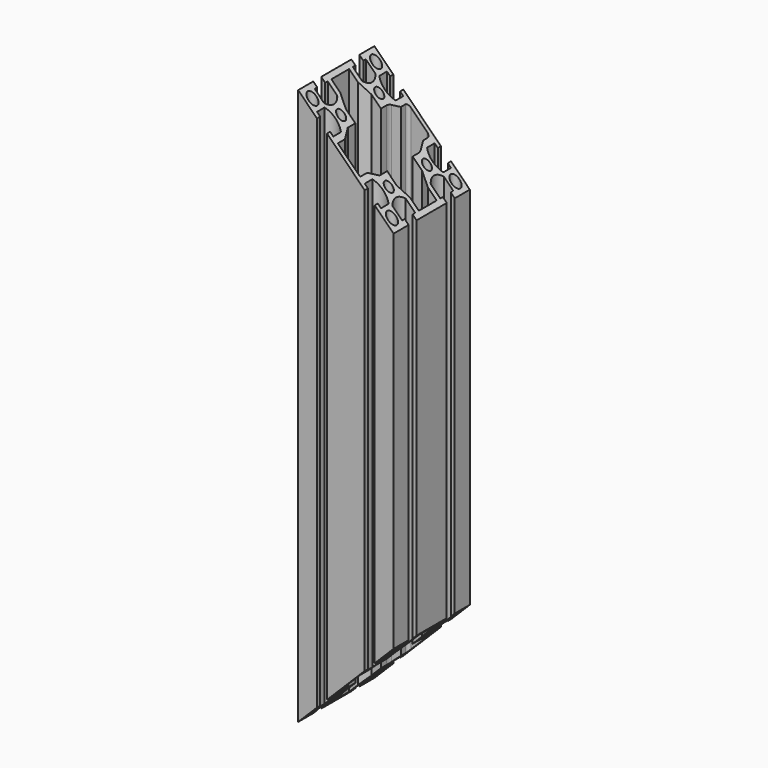
from build123d import *

# Parameters (mm, degrees)
F0_R     = 3
F0_R_2   = 2.5
F1_DEPTH = 350
F2_R     = 2
F3_R     = 7
F5_DEPTH = 60


# Not quite as in the source:
# - a feature names something its author has since deleted; it is built from what else it names


with BuildPart() as f1:
    # F0 (on Top) → F1 (new body)
    with BuildSketch(Plane.XY):
        with BuildLine():
            Line((18.15, -30), (30, -30))
            Line((30, -30), (30, -18.15))
            Line((30, -18.15), (27.5, -18.15))
            Line((27.5, -18.15), (27.5, -20.15))
            Line((27.5, -20.15), (21.5477069044, -20.15))
            ThreePointArc((21.5477069044, -20.15), (19.5, -15), (21.5477069044, -9.85))
            Line((21.5477069044, -9.85), (27.5, -9.85))
            Line((27.5, -9.85), (27.5, -11.85))
            Line((27.5, -11.85), (30, -11.85))
            Line((30, -11.85), (30, 11.85))
            Line((30, 11.85), (27.5, 11.85))
            Line((27.5, 11.85), (27.5, 9.85))
            Line((27.5, 9.85), (21.5477069044, 9.85))
            ThreePointArc((21.5477069044, 9.85), (19.5, 15), (21.5477069044, 20.15))
            Line((21.5477069044, 20.15), (27.5, 20.15))
            Line((27.5, 20.15), (27.5, 18.15))
            Line((27.5, 18.15), (30, 18.15))
            Line((30, 18.15), (30, 30))
            Line((30, 30), (18.15, 30))
            Line((18.15, 30), (18.15, 27.5))
            Line((18.15, 27.5), (20.15, 27.5))
            Line((20.15, 27.5), (20.15, 21.5477069044))
            ThreePointArc((20.15, 21.5477069044), (15, 19.5), (9.85, 21.5477069044))
            Line((9.85, 21.5477069044), (9.85, 27.5))
            Line((9.85, 27.5), (11.85, 27.5))
            Line((11.85, 27.5), (11.85, 30))
            Line((11.85, 30), (-11.85, 30))
            Line((-11.85, 30), (-11.85, 27.5))
            Line((-11.85, 27.5), (-9.85, 27.5))
            Line((-9.85, 27.5), (-9.85, 21.5477069044))
            ThreePointArc((-9.85, 21.5477069044), (-15, 19.5), (-20.15, 21.5477069044))
            Line((-20.15, 21.5477069044), (-20.15, 27.5))
            Line((-20.15, 27.5), (-18.15, 27.5))
            Line((-18.15, 27.5), (-18.15, 30))
            Line((-18.15, 30), (-30, 30))
            Line((-30, 30), (-30, 18.15))
            Line((-30, 18.15), (-27.5, 18.15))
            Line((-27.5, 18.15), (-27.5, 20.15))
            Line((-27.5, 20.15), (-21.5477069044, 20.15))
            ThreePointArc((-21.5477069044, 20.15), (-19.5, 15), (-21.5477069044, 9.85))
            Line((-21.5477069044, 9.85), (-27.5, 9.85))
            Line((-27.5, 9.85), (-27.5, 11.85))
            Line((-27.5, 11.85), (-30, 11.85))
            Line((-30, 11.85), (-30, -11.85))
            Line((-30, -11.85), (-27.5, -11.85))
            Line((-27.5, -11.85), (-27.5, -9.85))
            Line((-27.5, -9.85), (-21.5477069044, -9.85))
            ThreePointArc((-21.5477069044, -9.85), (-19.5, -15), (-21.5477069044, -20.15))
            Line((-21.5477069044, -20.15), (-27.5, -20.15))
            Line((-27.5, -20.15), (-27.5, -18.15))
            Line((-27.5, -18.15), (-30, -18.15))
            Line((-30, -18.15), (-30, -30))
            Line((-30, -30), (-18.15, -30))
            Line((-18.15, -30), (-18.15, -27.5))
            Line((-18.15, -27.5), (-20.15, -27.5))
            Line((-20.15, -27.5), (-20.15, -21.5477069044))
            ThreePointArc((-20.15, -21.5477069044), (-15, -19.5), (-9.85, -21.5477069044))
            Line((-9.85, -21.5477069044), (-9.85, -27.5))
            Line((-9.85, -27.5), (-11.85, -27.5))
            Line((-11.85, -27.5), (-11.85, -30))
            Line((-11.85, -30), (11.85, -30))
            Line((11.85, -30), (11.85, -27.5))
            Line((11.85, -27.5), (9.85, -27.5))
            Line((9.85, -27.5), (9.85, -21.5477069044))
            ThreePointArc((9.85, -21.5477069044), (15, -19.5), (20.15, -21.5477069044))
            Line((20.15, -21.5477069044), (20.15, -27.5))
            Line((20.15, -27.5), (18.15, -27.5))
            Line((18.15, -27.5), (18.15, -30))
        make_face()
        with Locations((-25, -25)):
            Circle(F0_R, mode=Mode.SUBTRACT)
        with Locations((-15, -15)):
            Circle(F0_R_2, mode=Mode.SUBTRACT)
        with Locations((25, -25)):
            Circle(F0_R, mode=Mode.SUBTRACT)
        with Locations((15, -15)):
            Circle(F0_R_2, mode=Mode.SUBTRACT)
        with Locations((-25, 25)):
            Circle(F0_R, mode=Mode.SUBTRACT)
        with Locations((-15, 15)):
            Circle(F0_R_2, mode=Mode.SUBTRACT)
        Polygon((-7, 22), (-7, 27.5), (0, 27.5), (7, 27.5), (7, 22), (10, 16), (10, 10), (16, 10), (22, 7), (27.5, 7), (27.5, 0), (27.5, -7), (22, -7), (16, -10), (10, -10), (10, -16), (7, -22), (7, -27.5), (0, -27.5), (-7, -27.5), (-7, -22), (-10, -16), (-10, -10), (-16, -10), (-22, -7), (-27.5, -7), (-27.5, 0), (-27.5, 7), (-22, 7), (-16, 10), (-10, 10), (-10, 16), align=None, mode=Mode.SUBTRACT)
        with Locations((15, 15)):
            Circle(F0_R_2, mode=Mode.SUBTRACT)
        with Locations((25, 25)):
            Circle(F0_R, mode=Mode.SUBTRACT)
    extrude(amount=F1_DEPTH)

    # F2
    f2_edges = [f1.edges().sort_by_distance(p)[0] for p in [
        (-7, 27.5, 175),
        (7, 27.5, 175),
    ]]
    fillet(f2_edges, radius=F2_R)

    # F3
    f3_edges = [f1.edges().sort_by_distance(p)[0] for p in [
        (-10, 16, 175),
        (10, 16, 175),
    ]]
    fillet(f3_edges, radius=F3_R)

    # F4 (on face) → F5 (cut)
    with BuildSketch(Plane.XZ.offset(30)):
        Polygon((30, 0), (30, 60), (-30, 0), (-18.15, 0), align=None)
        Polygon((30, 290), (30, 350), (-18.15, 350), (-30, 350), align=None)
    extrude(amount=-F5_DEPTH, mode=Mode.SUBTRACT)


solid = f1.part
